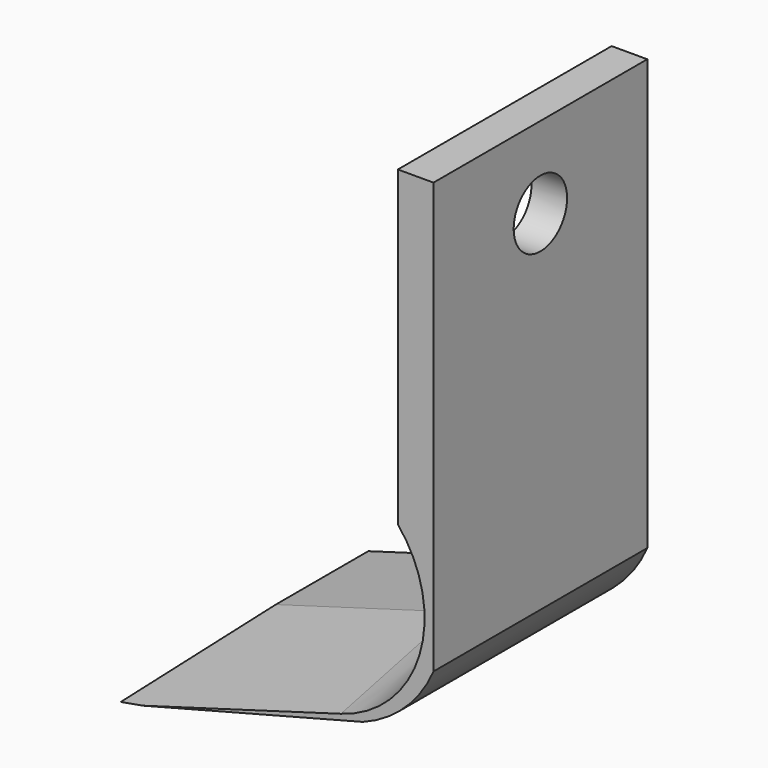
from build123d import *

# Parameters (mm, degrees)
F1_DEPTH    = 60
F2_T1_DEPTH = 130.2639714598
F2_T4_ANGLE = 327.2570469478
F3_R        = 7.5
F4_DEPTH    = 25


# Not quite as in the source:
# - a fillet or chamfer that OpenCascade refuses, or shapes differently, is made with other operations: its cross-section is extruded or revolved along the edge and cut away or added


with BuildPart() as f1:
    # F0 (on Front) → F1 (new body)
    with BuildSketch(Plane.XZ):
        with BuildLine():
            Line((15.8661792875, 46.7765345339), (7.8661792875, 46.7765345339))
            Line((7.8661792875, 46.7765345339), (7.8661792875, -40.0019907292))
            ThreePointArc((7.8661792875, -40.0019907292), (3.8517652045, -52.021185498), (-6.5799250014, -59.2153777921))
            Line((-6.5799250014, -59.2153777921), (-46.7759604719, -70.834598717))
            Line((-46.7759604719, -70.834598717), (-55.08180854, -79.3164507385))
            Line((-55.08180854, -79.3164507385), (0, -64.9890005589))
            ThreePointArc((0, -64.9890005589), (9.4773105279, -59.0361843334), (15.8661792875, -49.8471804794))
            Line((15.8661792875, -49.8471804794), (15.8661792875, -40.0019907292))
            Line((15.8661792875, -40.0019907292), (15.8661792875, 46.7765345339))
        make_face()
    extrude(amount=F1_DEPTH)

    # F2: chamfer of 6 x 34.0276909177 on 2 edges, made by hand

    # F2_s2 → F2_t1 (cut)
    with BuildSketch(Plane(origin=(-21.8695743552, 0, -6.3217034464), x_dir=(0, 1, 0), z_dir=(-0.9606693531, 0, -0.2776947856))):
        Polygon((-60, 61.0591878178), (-25.9723090823, 55.0591878178), (-60, 55.0591878178), align=None)
    extrude(amount=F2_T1_DEPTH, mode=Mode.SUBTRACT)

    # F2_s3 → F2_t4 (revolve, cut)
    with BuildSketch(Plane(origin=(-0.1774752696, 0, 0.0529760926), x_dir=(0, 1, 0), z_dir=(0.9582213809, 0, -0.2860275953))):
        Polygon((-60, -67.8013703537), (-25.9723090823, -61.8013703537), (-60, -61.8013703537), align=None)
    revolve(axis=Axis((-12.1338207125, -60, -40.0019907292), (0, 1, 0)), revolution_arc=F2_T4_ANGLE, mode=Mode.SUBTRACT)

    # F3 (on face) → F4 (cut)
    with BuildSketch(Plane(origin=(7.8661792875, 0, 0), x_dir=(0, -1, 0), z_dir=(-1, 0, 0))):
        with Locations((30, 28.4848585725)):
            Circle(F3_R)
    extrude(amount=-F4_DEPTH, mode=Mode.SUBTRACT)


solid = f1.part
